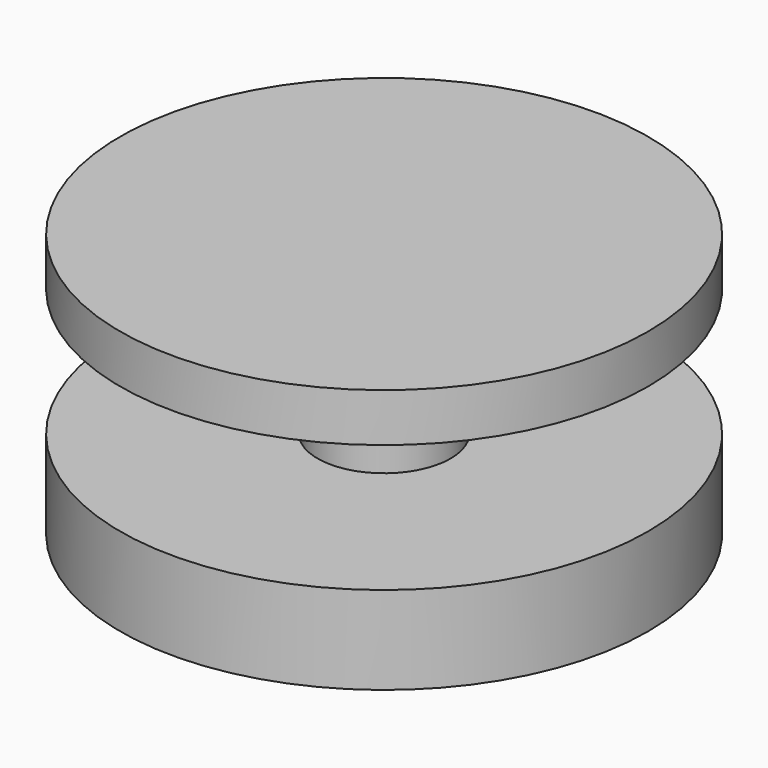
from build123d import *

# Parameters (mm, degrees)
F0_R      = 120
F0_R_2    = 100
F1_DEPTH  = 9
F2_DEPTH  = 4
F3_DEPTH  = 13
F4_DEPTH  = 9
F5_R      = 30.25
F6_DEPTH  = 58
F7_START  = -80
F4_FACE_R = 120
F7_DEPTH  = 40
F8_START  = 73
F5_R_2    = 80
F8_DEPTH  = 25


with BuildPart() as f1:
    # F0 (on Top) → F1 (new body)
    with BuildSketch(Plane.XY):
        Circle(F0_R)
        Circle(F0_R_2, mode=Mode.SUBTRACT)
        Circle(F0_R_2)
    extrude(amount=-F1_DEPTH)

    # F0 (on Top) → F3 (join)
    with BuildSketch(Plane.XY):
        Circle(F0_R)
        Circle(F0_R_2, mode=Mode.SUBTRACT)
    extrude(amount=F3_DEPTH)



with BuildPart() as f2:
    # F0 (on Top) → F2 (new body)
    with BuildSketch(Plane.XY):
        Circle(F0_R_2)
    extrude(amount=F2_DEPTH)


with BuildPart() as f1_1:
    add(f1.part)
    # F4 (add): a face of the model
    f4_faces = [f2.part.faces().sort_by_distance(p)[0] for p in [
        (0, 0, 4),
    ]]
    extrude(f4_faces, amount=F4_DEPTH)

    # F5 (on face) → F6 (join)
    with BuildSketch(Plane(origin=(0, 0, -9), x_dir=(1, 0, 0), z_dir=(0, 0, -1))):
        Circle(F5_R)
    extrude(amount=F6_DEPTH)

    # F4_face (on face) → F7 (join)
    with BuildSketch(Plane.XY.offset(13).offset(F7_START)):
        Circle(F4_FACE_R)
    extrude(amount=-F7_DEPTH)

    # F5 (on face) → F8 (cut)
    with BuildSketch(Plane(origin=(0, 0, -9), x_dir=(1, 0, 0), z_dir=(0, 0, -1)).offset(F8_START)):
        Circle(F5_R_2)
        Circle(F5_R, mode=Mode.SUBTRACT)
        Circle(F5_R)
    extrude(amount=F8_DEPTH, mode=Mode.SUBTRACT)


solid = Compound([f2.part, f1_1.part])
